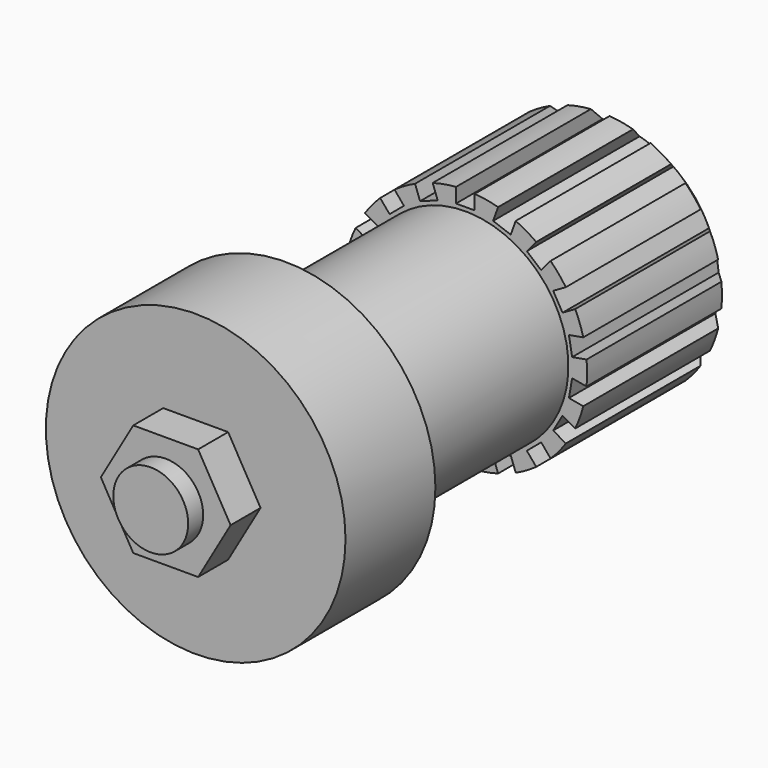
from build123d import *

# Parameters (mm, degrees)
F0_R             = 8
F1_DEPTH         = 6
F3_DEPTH         = 2
F4_R             = 2
F5_DEPTH         = 1
F6_R             = 5.5
F7_DEPTH         = 22
F8_R             = 6.5
F8_R_2           = 5.5
F9_DEPTH         = 10
F10_SIZE         = 1
F11_W            = 1
F11_H            = 2
F12_DEPTH        = 20
F12_COPIES_COUNT = 18


# Not quite as in the source:
# - a pattern or mirror of a feature is missing from the dataset's text; its kind, count and spacing are read off the source's solid


with BuildPart() as f1:
    # F0 (on Front) → F1 (new body)
    with BuildSketch(Plane.XZ):
        Circle(F0_R)
    extrude(amount=-F1_DEPTH)

    # F2 (on face) → F3 (join)
    with BuildSketch(Plane.XZ):
        Polygon((1.7320508076, -3), (3.4641016151, 0), (1.7320508076, 3), (-1.7320508076, 3), (-3.4641016151, 0), (-1.7320508076, -3), align=None)
    extrude(amount=F3_DEPTH)

    # F4 (on face) → F5 (join)
    with BuildSketch(Plane.XZ.offset(2)):
        Circle(F4_R)
    extrude(amount=F5_DEPTH)

    # F6 (on face) → F7 (join)
    with BuildSketch(Plane(origin=(0, 6, 0), x_dir=(-1, 0, 0), z_dir=(0, 1, 0))):
        Circle(F6_R)
    extrude(amount=F7_DEPTH)

    # F8 (on face) → F9 (join)
    with BuildSketch(Plane(origin=(0, 28, 0), x_dir=(-1, 0, 0), z_dir=(0, 1, 0))):
        Circle(F8_R)
        Circle(F8_R_2, mode=Mode.SUBTRACT)
    extrude(amount=-F9_DEPTH)

    # F10
    f10_edges = [f1.edges().sort_by_distance(p)[0] for p in [
        (6.5, 28, 0),
    ]]
    chamfer(f10_edges, length=F10_SIZE)

    # F11 (on face) → F12 (cut)
    with BuildSketch(Plane(origin=(0, 28, 0), x_dir=(-1, 0, 0), z_dir=(0, 1, 0))):
        with Locations((0, 6.7)):
            Rectangle(F11_W, F11_H)
    f12 = extrude(amount=-F12_DEPTH, mode=Mode.SUBTRACT)

    # F12_copies: F12 ×18 about axis
    f12_copies_axis = Axis((0, 0, 0), (0, 1, 0))
    for i in range(1, F12_COPIES_COUNT):
        add(f12.rotate(f12_copies_axis, i * 360 / F12_COPIES_COUNT), mode=Mode.SUBTRACT)


solid = f1.part
